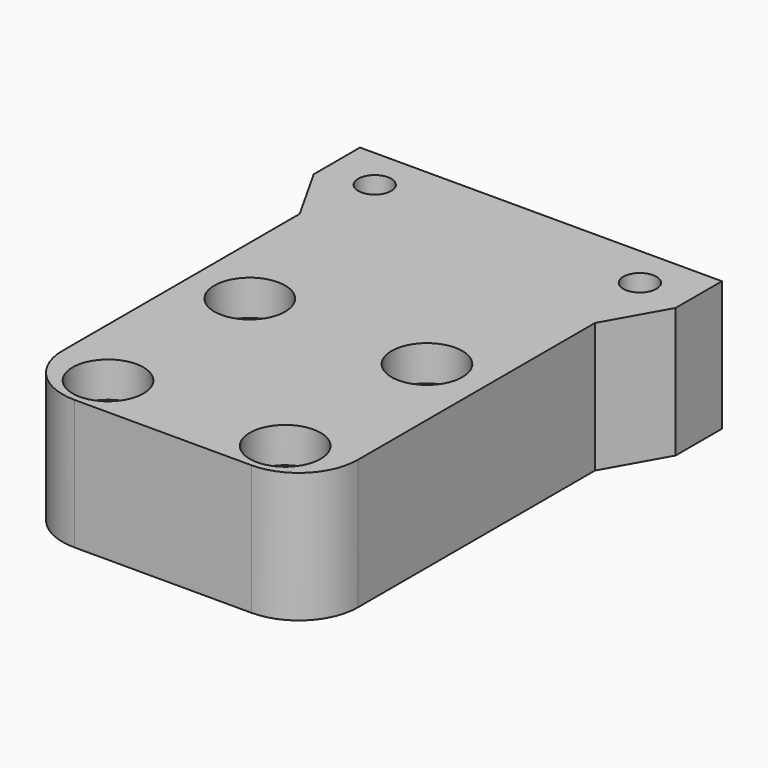
from build123d import *

# Parameters (mm, degrees)
F0_W     = 25
F0_H     = 30.0927665085
F0_W_2   = 30.6387297809
F0_H_2   = 4.8959264159
F1_DEPTH = 11
F2_R     = 1.675
F3_DEPTH = 25
F4_R     = 5
F5_DEPTH = 11
F6_R     = 1.4
F7_DEPTH = 11.001
F2_R_2   = 3
F8_DEPTH = 3


# Not quite as in the source:
# - a feature names something its author has since deleted; it is built from what else it names


with BuildPart() as f1:
    # F0 (on Top) → F1 (new body)
    with BuildSketch(Plane.XY):
        with Locations((12.5, 15.0463832542)):
            Rectangle(F0_W, F0_H)
        Polygon((-2.8193648905, 35.1040735841), (0, 30.0927665085), (25, 30.0927665085), (27.8193648905, 35.1040735841), align=None)
        with Locations((12.5, 37.552036792)):
            Rectangle(F0_W_2, F0_H_2)
    extrude(amount=F1_DEPTH)

    # F2 (on face) → F3 (cut)
    with BuildSketch(Plane.XY.offset(11)):
        with BuildLine():
            ThreePointArc((3.325, 18.5605346784), (5, 16.8855346784), (6.675, 18.5605346784))
            ThreePointArc((6.675, 18.5605346784), (5, 20.2355346784), (3.325, 18.5605346784))
        make_face()
        with Locations((20, 18.5605346784)):
            Circle(F2_R)
        with Locations((20, 3.5605346784)):
            Circle(F2_R)
        with Locations((5, 3.5605346784)):
            Circle(F2_R)
    extrude(amount=-F3_DEPTH, mode=Mode.SUBTRACT)

    # F4
    f4_edges = [f1.edges().sort_by_distance(p)[0] for p in [
        (0, 0, 5.5),
        (25, 0, 5.5),
    ]]
    fillet(f4_edges, radius=F4_R)

    # F0 (on Top) → F5 (join)
    with BuildSketch(Plane.XY):
        with Locations((12.5, 37.552036792)):
            Rectangle(F0_W_2, F0_H_2)
        Polygon((-2.8193648905, 35.1040735841), (0, 30.0927665085), (25, 30.0927665085), (27.8193648905, 35.1040735841), align=None)
    extrude(amount=F5_DEPTH)

    # F6 (on face) → F7 (cut, through all)
    with BuildSketch(Plane.XY.offset(11)):
        with Locations((23.7225, 36.4378243685)):
            Circle(F6_R)
        with BuildLine():
            ThreePointArc((-0.1225, 36.4378243685), (1.2775, 35.0378243685), (2.6775, 36.4378243685))
            ThreePointArc((2.6775, 36.4378243685), (1.2775, 37.8378243685), (-0.1225, 36.4378243685))
        make_face()
    extrude(amount=-F7_DEPTH, mode=Mode.SUBTRACT)

    # F2 (on face) → F8 (cut)
    with BuildSketch(Plane.XY.offset(11)):
        with BuildLine():
            ThreePointArc((8, 18.5605346784), (5, 21.5605346784), (2, 18.5605346784))
            ThreePointArc((2, 18.5605346784), (5, 15.5605346784), (8, 18.5605346784))
        make_face()
        with BuildLine():
            ThreePointArc((3.325, 18.5605346784), (5, 20.2355346784), (6.675, 18.5605346784))
            ThreePointArc((6.675, 18.5605346784), (5, 16.8855346784), (3.325, 18.5605346784))
        make_face(mode=Mode.SUBTRACT)
        with Locations((5, 3.5605346784)):
            Circle(F2_R_2)
        with Locations((5, 3.5605346784)):
            Circle(F2_R, mode=Mode.SUBTRACT)
        with Locations((20, 18.5605346784)):
            Circle(F2_R_2)
        with Locations((20, 18.5605346784)):
            Circle(F2_R, mode=Mode.SUBTRACT)
        with Locations((20, 3.5605346784)):
            Circle(F2_R_2)
        with Locations((20, 3.5605346784)):
            Circle(F2_R, mode=Mode.SUBTRACT)
    extrude(amount=-F8_DEPTH, mode=Mode.SUBTRACT)


solid = f1.part
